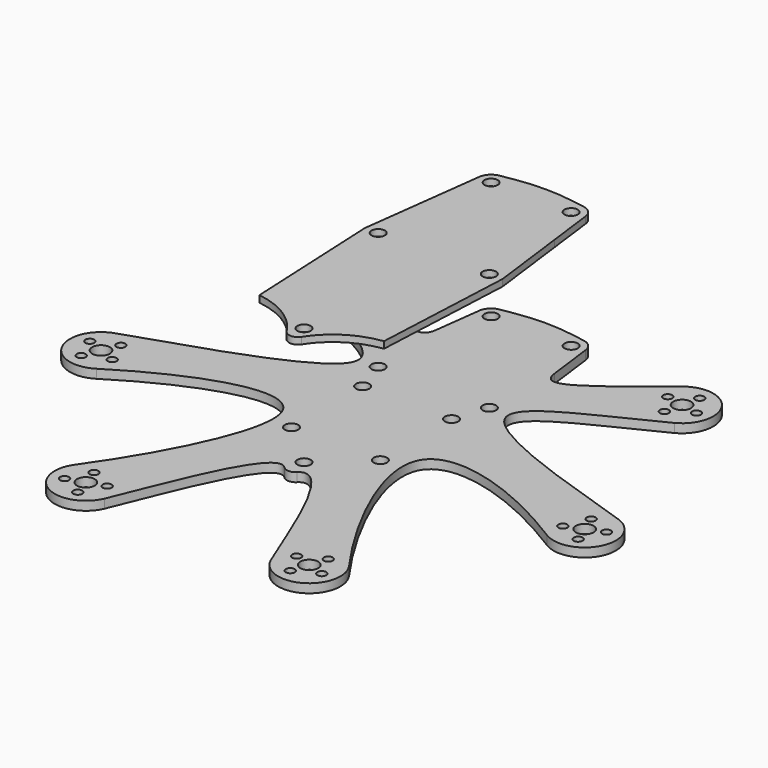
from build123d import *
from build123d import SkipClean  # not in build123d's __all__

# Parameters (mm, degrees)
F0_R     = 1
F0_R_2   = 2
F0_R_3   = 1.5
F1_DEPTH = 2
F3_START = 27
F3_DEPTH = 1.5
F5_R     = 2
F5_2_R   = 2
F6_R     = 40
F6_2_R   = 40


with BuildPart() as f1:
    # F0 (on Top) → F1 (new body)
    with BuildSketch(Plane.XY):
        with BuildLine():
            ThreePointArc((-41.4963104591, 33.3223288889), (-34.6244361147, 33.5340840773), (-31.24818631, 39.523110252))
            ThreePointArc((-31.24818631, 39.523110252), (-31.9341865743, 42.5452630174), (-33.8577312636, 44.9750736126))
            ThreePointArc((-33.8577312636, 44.9750736126), (-44.1024877089, 43.3607078249), (-41.4963104591, 33.3223288889))
        make_face()
        with Locations((-37.3937638756, 35.6154303389)):
            Circle(F0_R, mode=Mode.SUBTRACT)
        with Locations((-42.1558662232, 38.6686878176)):
            Circle(F0_R, mode=Mode.SUBTRACT)
        with Locations((-38.24818631, 39.523110252)):
            Circle(F0_R_2, mode=Mode.SUBTRACT)
        with Locations((-39.1026087444, 43.4307901652)):
            Circle(F0_R, mode=Mode.SUBTRACT)
        with Locations((-34.3405063969, 40.3775326864)):
            Circle(F0_R, mode=Mode.SUBTRACT)
        with BuildLine():
            ThreePointArc((-47.4048499874, -8.0692191595), (-50.4343142983, -2.3042520008), (-56.9005203707, -1.5292169166))
            ThreePointArc((-56.9005203707, -1.5292169166), (-60.6686355635, -11.194117599), (-50.6808388136, -13.9964226129))
            ThreePointArc((-50.6808388136, -13.9964226129), (-48.2783469793, -11.455361639), (-47.4048499874, -8.0692191595))
        make_face()
        with Locations((-55.9046783302, -11.7773878372)):
            Circle(F0_R, mode=Mode.SUBTRACT)
        with Locations((-58.1130186652, -6.5693908168)):
            Circle(F0_R, mode=Mode.SUBTRACT)
        with Locations((-54.4048499874, -8.0692191595)):
            Circle(F0_R_2, mode=Mode.SUBTRACT)
        with Locations((-50.6966813097, -9.5690475022)):
            Circle(F0_R, mode=Mode.SUBTRACT)
        with Locations((-52.9050216447, -4.3610504818)):
            Circle(F0_R, mode=Mode.SUBTRACT)
        with BuildLine():
            ThreePointArc((-18.13, -48.9232368103), (-22.990524377, -42.2582053731), (-30.8221840168, -44.8490447286))
            ThreePointArc((-30.8221840168, -44.8490447286), (-28.5810959404, -55.0133876139), (-18.7098219402, -51.7127374251))
            ThreePointArc((-18.7098219402, -51.7127374251), (-18.2764882571, -50.3477987748), (-18.13, -48.9232368103))
        make_face()
        with Locations((-28.9382578849, -50.1468265627)):
            Circle(F0_R, mode=Mode.SUBTRACT)
        with Locations((-23.9064102476, -52.7314946952)):
            Circle(F0_R, mode=Mode.SUBTRACT)
        with Locations((-26.3535897524, -45.1149789254)):
            Circle(F0_R, mode=Mode.SUBTRACT)
        with Locations((-25.13, -48.9232368103)):
            Circle(F0_R_2, mode=Mode.SUBTRACT)
        with Locations((-21.3217421151, -47.699647058)):
            Circle(F0_R, mode=Mode.SUBTRACT)
        with BuildLine():
            ThreePointArc((-33.8577312636, 44.9750736126), (-31.9341865743, 42.5452630174), (-31.24818631, 39.523110252))
            ThreePointArc((-31.24818631, 39.523110252), (-34.6244361147, 33.5340840773), (-41.4963104591, 33.3223288889))
            add(Edge.make_bspline(
                [(-56.9005203707, -1.5292169166), (-50.3186728015, 0.9824216786), (2.6616248501, 15.4386103021), (-27.894211933, 26.1972099543), (-41.4963104591, 33.3223288889)],
                knots=[0, 0, 0, 0, 0.5455847742, 1, 1, 1, 1], degree=3))
            ThreePointArc((-56.9005203707, -1.5292169166), (-50.4343142983, -2.3042520008), (-47.4048499874, -8.0692191595))
            ThreePointArc((-47.4048499874, -8.0692191595), (-48.2783469793, -11.455361639), (-50.6808388136, -13.9964226129))
            add(Edge.make_bspline(
                [(-50.6808388136, -13.9964226129), (-33.8360257447, -3.4129708074), (-2.4373665833, 5.0967457749), (-21.6071682121, -31.974451527), (-30.8221840168, -44.8490447286)],
                knots=[0, 0, 0, 0, 0.481713355, 1, 1, 1, 1], degree=3))
            ThreePointArc((-30.8221840168, -44.8490447286), (-22.990524377, -42.2582053731), (-18.13, -48.9232368103))
            ThreePointArc((-18.13, -48.9232368103), (-18.2764882571, -50.3477987748), (-18.7098219402, -51.7127374251))
            add(Edge.make_bspline(
                [(-18.7098219402, -51.7127374251), (-14.7297938944, -42.5524997105), (-4.2223660275, -11.9342948571), (0, -25.5)],
                knots=[0, 0, 0, 0, 32.2050468149, 32.2050468149, 32.2050468149, 32.2050468149], degree=3))
            add(Edge.make_bspline(
                [(-14.0167400241, -14.0061862767), (-5.1296344027, -15.2601953596), (-0.9314316558, -21.8573715538), (0, -25.5)],
                knots=[0, 0, 0, 0, 18.1266862611, 18.1266862611, 18.1266862611, 18.1266862611], degree=3))
            Line((-14.0167400241, -14.0061862767), (-15.5, 17.5))
            Line((-15.5, 17.5), (-13.2968256499, 34.8553436253))
            add(Edge.make_bspline(
                [(-33.8577312636, 44.9750736126), (-20.1089866459, 33.9032374322), (-14.0507456444, 28.9163944135), (-13.2968256499, 34.8553436253)],
                knots=[0, 0, 0, 0, 22.9163647786, 22.9163647786, 22.9163647786, 22.9163647786], degree=3))
        make_face()
        with BuildLine():
            Line((-11.9761157322, 45.2591386998), (-13.2968256499, 34.8553436253))
            Line((-13.2968256499, 34.8553436253), (-15.5, 17.5))
            Line((-15.5, 17.5), (-14.0167400241, -14.0061862767))
            add(Edge.make_bspline(
                [(-14.0167400241, -14.0061862767), (-5.1296344027, -15.2601953596), (-0.9314316558, -21.8573715538), (0, -25.5)],
                knots=[0, 0, 0, 0, 18.1266862611, 18.1266862611, 18.1266862611, 18.1266862611], degree=3))
            Line((0, -25.5), (0, -20.490599284))
            ThreePointArc((0, -20.490599284), (-1.5, -18.990599284), (0, -17.490599284))
            Line((0, -17.490599284), (0, 49.3813356447))
            Line((0, 49.3813356447), (-9.4806248475, 47.8425853396))
            ThreePointArc((-9.4806248475, 47.8425853396), (-11.1577333, 46.9656069816), (-11.9761157322, 45.2591386998))
        make_face()
        with Locations((-10, -10)):
            Circle(F0_R_3, mode=Mode.SUBTRACT)
        with Locations((-10, 10)):
            Circle(F0_R_3, mode=Mode.SUBTRACT)
        with Locations((-12.5, 17.5)):
            Circle(F0_R_3, mode=Mode.SUBTRACT)
        with Locations((-9, 44.8813356447)):
            Circle(F0_R_3, mode=Mode.SUBTRACT)
    extrude(amount=F1_DEPTH)

    # F2: F1 across face


with BuildPart() as f1_1:
    add(f1.part, clean=False)
    with SkipClean():  # cleaning this boolean's faces spoils the solid; the shape is the same uncleaned
        add(f1.part.mirror(Plane(origin=(0, 15.9453681803, 1), x_dir=(0, 1, 0), z_dir=(1, 0, 0))), clean=False)

    # F5
    f5_edges = [f1_1.edges().sort_by_distance(p)[0] for p in [
        (0, -25.5, 1),
    ]]
    fillet(f5_edges, radius=F5_R)

    # F6
    f6_edges = [f1_1.edges().sort_by_distance(p)[0] for p in [
        (0, 49.381336, 1),
    ]]
    fillet(f6_edges, radius=F6_R)


with BuildPart() as f3:
    # F0 (on Top) → F3 (new body)
    with BuildSketch(Plane.XY.offset(F3_START)):
        with BuildLine():
            Line((-11.9761157322, 45.2591386998), (-13.2968256499, 34.8553436253))
            Line((-13.2968256499, 34.8553436253), (-15.5, 17.5))
            Line((-15.5, 17.5), (-14.0167400241, -14.0061862767))
            add(Edge.make_bspline(
                [(-14.0167400241, -14.0061862767), (-5.1296344027, -15.2601953596), (-0.9314316558, -21.8573715538), (0, -25.5)],
                knots=[0, 0, 0, 0, 18.1266862611, 18.1266862611, 18.1266862611, 18.1266862611], degree=3))
            Line((0, -25.5), (0, -20.490599284))
            ThreePointArc((0, -20.490599284), (-1.5, -18.990599284), (0, -17.490599284))
            Line((0, -17.490599284), (0, 49.3813356447))
            Line((0, 49.3813356447), (-9.4806248475, 47.8425853396))
            ThreePointArc((-9.4806248475, 47.8425853396), (-11.1577333, 46.9656069816), (-11.9761157322, 45.2591386998))
        make_face()
        with Locations((-10, -10)):
            Circle(F0_R_3, mode=Mode.SUBTRACT)
        with Locations((-10, 10)):
            Circle(F0_R_3, mode=Mode.SUBTRACT)
        with Locations((-12.5, 17.5)):
            Circle(F0_R_3, mode=Mode.SUBTRACT)
        with Locations((-9, 44.8813356447)):
            Circle(F0_R_3, mode=Mode.SUBTRACT)
        with Locations((-10, -10)):
            Circle(F0_R_3)
        with Locations((-10, 10)):
            Circle(F0_R_3)
    extrude(amount=F3_DEPTH)

    # F4: F3 across face


with BuildPart() as f3_1:
    add(f3.part, clean=False)
    with SkipClean():  # cleaning this boolean's faces spoils the solid; the shape is the same uncleaned
        add(f3.part.mirror(Plane(origin=(0, 15.9453681803, 27.75), x_dir=(0, 1, 0), z_dir=(1, 0, 0))), clean=False)

    # F5#2
    f5_2_edges = [f3_1.edges().sort_by_distance(p)[0] for p in [
        (0, -25.5, 27.75),
    ]]
    fillet(f5_2_edges, radius=F5_2_R)

    # F6#2
    f6_2_edges = [f3_1.edges().sort_by_distance(p)[0] for p in [
        (0, 49.381336, 27.75),
    ]]
    fillet(f6_2_edges, radius=F6_2_R)


solid = Compound([f1_1.part, f3_1.part])
